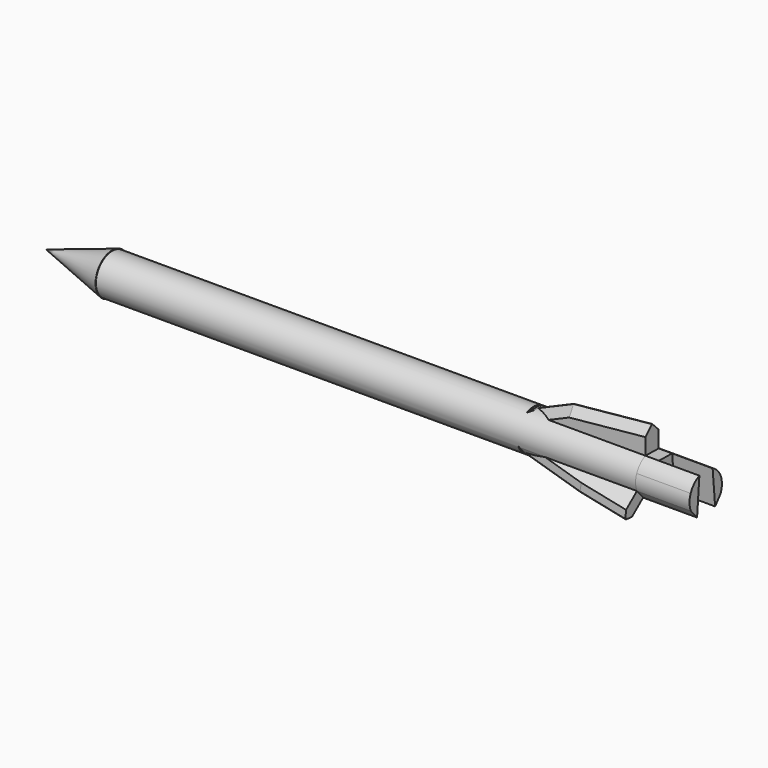
from build123d import *

# Parameters (mm, degrees)
F0_R          = 9.525
F1_DEPTH      = 254
F5_DEPTH      = 55.626
F7_DEPTH      = 6.35
F8_DEPTH      = 25.4
F10_DEPTH     = 25.4
F12_DEPTH     = 25.4
F14_DEPTH     = 25.4
F15_T1_DEPTH  = 44.8533405939
F15_T3_DEPTH  = 44.8533405939
F15_T8_DEPTH  = 28.2795963183
F15_S9_R      = 9.525
F15_T10_DEPTH = 17
F15_T14_DEPTH = 27.9095113127
F15_S15_R     = 9.525
F15_T16_DEPTH = 17
F16_T1_DEPTH  = 52.8359208118
F16_T3_DEPTH  = 52.8359208118
F16_T8_DEPTH  = 31.126263523
F16_S9_R      = 9.525
F16_T10_DEPTH = 18
F16_T14_DEPTH = 35.8525293061
F16_S15_R     = 9.525
F16_T16_DEPTH = 20
F17_T1_DEPTH  = 37.2074314298
F17_T3_DEPTH  = 37.2074314298
F17_T8_DEPTH  = 45.6448991689
F17_S9_R      = 9.525
F17_T10_DEPTH = 25
F17_T14_DEPTH = 44.9174010309
F17_S15_R     = 9.525
F17_T16_DEPTH = 25


# Not quite as in the source:
# - a fillet or chamfer that OpenCascade refuses, or shapes differently, is made with other operations: its cross-section is extruded or revolved along the edge and cut away or added
# - a feature names something its author has since deleted; it is built from what else it names


with BuildPart() as f1:
    # F0 (on Right) → F1 (new body)
    with BuildSketch(Plane.YZ):
        Circle(F0_R)
    extrude(amount=F1_DEPTH)

    # F2 (on Front) → F3 (revolve)
    with BuildSketch(Plane.XZ):
        Polygon((0, -9.7508067265), (0, 0), (-31.0870110989, 0), align=None)
    revolve(axis=Axis((-15.5435055494, 0, 0), (-1, 0, 0)))

    # F4 (on face) → F5 (join)
    with BuildSketch(Plane.YZ.offset(254)):
        with BuildLine():
            ThreePointArc((-3.7328505423, 8.7630731955), (0.1780475173, 9.5233357644), (4.0577948396, 8.6174199178))
            Line((4.0577948396, 8.6174199178), (4.0577948396, 20.311106017))
            Line((4.0577948396, 20.311106017), (-3.7328505423, 20.311106017))
            Line((-3.7328505423, 20.311106017), (-3.7328505423, 8.7630731955))
        make_face()
        with BuildLine():
            ThreePointArc((-5.0939482873, -8.0484356149), (-7.2224802699, -6.2097829069), (-8.7212105654, -3.8296359191))
            Line((-8.7212105654, -3.8296359191), (-17.1272028238, -10.6496075168))
            Line((-17.1272028238, -10.6496075168), (-13.6232364185, -14.9684399422))
            Line((-13.6232364185, -14.9684399422), (-5.0939482873, -8.0484356149))
        make_face()
        with BuildLine():
            Line((13.9740978255, -12.0467544007), (8.7309135752, -3.8074628223))
            ThreePointArc((8.7309135752, -3.8074628223), (7.3970545146, -6.0007674099), (5.5259177996, -7.75821226))
            Line((5.5259177996, -7.75821226), (9.9034377135, -14.6371738298))
            Line((9.9034377135, -14.6371738298), (13.9740978255, -12.0467544007))
        make_face()
    extrude(amount=-F5_DEPTH)

    # F6 (on face) → F7 (join)
    with BuildSketch(Plane.YZ.offset(254)):
        Polygon((4.0577948396, 8.6174199178), (-3.7328505423, 8.7630731955), (-5.0939482873, -8.0484356149), (5.5259177996, -7.75821226), align=None)
        with BuildLine():
            Line((5.5259177996, -7.75821226), (-5.0939482873, -8.0484356149))
            ThreePointArc((-5.0939482873, -8.0484356149), (0.2602053301, -9.5214451732), (5.5259177996, -7.75821226))
        make_face()
    extrude(amount=F7_DEPTH)

    # F6 (on face) → F8 (join)
    with BuildSketch(Plane.YZ.offset(254)):
        Polygon((-5.0939482873, -8.0484356149), (-3.7328505423, 8.7630731955), (-8.8555062097, 3.5079388207), (-8.7212105654, -3.8296359191), align=None)
        Polygon((8.7309135752, 3.8074628223), (4.0577948396, 8.6174199178), (5.5259177996, -7.75821226), (8.7309135752, -3.8074628223), align=None)
        with BuildLine():
            ThreePointArc((9.525, 0), (9.3243653083, 1.9446944743), (8.7309135752, 3.8074628223))
            Line((8.7309135752, 3.8074628223), (8.7309135752, -3.8074628223))
            ThreePointArc((8.7309135752, -3.8074628223), (9.3243653083, -1.9446944743), (9.525, 0))
        make_face()
        with BuildLine():
            ThreePointArc((8.7309135752, 3.8074628223), (6.8316679914, 6.6373140242), (4.0577948396, 8.6174199178))
            Line((4.0577948396, 8.6174199178), (8.7309135752, 3.8074628223))
        make_face()
        with BuildLine():
            Line((-8.7212105654, -3.8296359191), (-8.8555062097, 3.5079388207))
            ThreePointArc((-8.8555062097, 3.5079388207), (-9.5234050588, -0.1743017091), (-8.7212105654, -3.8296359191))
        make_face()
        with BuildLine():
            Line((-8.8555062097, 3.5079388207), (-3.7328505423, 8.7630731955))
            ThreePointArc((-3.7328505423, 8.7630731955), (-6.8206151301, 6.6486716152), (-8.8555062097, 3.5079388207))
        make_face()
    extrude(amount=F8_DEPTH)

    # F9 (on face) → F10 (cut)
    with BuildSketch(Plane(origin=(0, 4.0577948396, 0), x_dir=(-1, 0, 0), z_dir=(0, 1, 0))):
        Polygon((-217.1654254198, 16.6623666883), (-198.374, 8.6174199178), (-198.374, 20.311106017), (-254, 20.311106017), align=None)
    extrude(amount=-F10_DEPTH, mode=Mode.SUBTRACT)

    # F11 (on face) → F12 (cut)
    with BuildSketch(Plane(origin=(0, 4.4898005119, 2.8571450721), x_dir=(-1, 0, 0), z_dir=(0, 0.843661548, 0.5368753975))):
        Polygon((-198.374, -7.8996226746), (-217.1549183124, -14.7158552648), (-254, -17.6657327906), (-198.374, -17.6657327906), align=None)
    extrude(amount=-F12_DEPTH, mode=Mode.SUBTRACT)

    # F13 (on face) → F14 (cut)
    with BuildSketch(Plane(origin=(0, 1.9157700793, -2.3612925984), x_dir=(1, 0, 0), z_dir=(0, 0.6300417268, -0.7765612806))):
        Polygon((230.1693707705, 16.137143597), (254, 20.0100196673), (198.374, 20.0100196673), (198.374, 9.0266132778), align=None)
    extrude(amount=-F14_DEPTH, mode=Mode.SUBTRACT)

    # F15: chamfer of 3.81 on 4 edges, made by hand

    # F15_s2 → F15_t1 (cut)
    with BuildSketch(Plane(origin=(257.4244465349, 0, 25.499811331), x_dir=(0, 1, 0), z_dir=(-0.9951296233, 0, -0.098575011))):
        with BuildLine():
            Line((0.1400317661, 4.7181064364), (4.165557913, 8.7436325833))
            Line((4.165557913, 8.7436325833), (4.241757913, 8.7436325833))
            ThreePointArc((4.241757913, 8.7436325833), (4.1339948396, 6.7847510466), (4.1339948396, 4.8258695099))
            Line((4.1339948396, 4.8258695099), (4.0577948396, 4.7496695099))
            ThreePointArc((4.0577948396, 4.7496695099), (2.0989133028, 4.7496695099), (0.1400317661, 4.6419064364))
            Line((0.1400317661, 4.6419064364), (0.1400317661, 4.7181064364))
        make_face()
    extrude(amount=F15_T1_DEPTH, mode=Mode.SUBTRACT)

    # F15_s4 → F15_t3 (cut)
    with BuildSketch(Plane(origin=(212.789558605, 0, 21.0783927893), x_dir=(0, 1, 0), z_dir=(0.9951296233, 0, 0.098575011))):
        with BuildLine():
            Line((-3.8406136157, -8.7436325833), (0.1849125312, -4.7181064364))
            Line((0.1849125312, -4.7181064364), (0.1849125312, -4.6419064364))
            ThreePointArc((0.1849125312, -4.6419064364), (-1.7739690056, -4.7496695099), (-3.7328505423, -4.7496695099))
            Line((-3.7328505423, -4.7496695099), (-3.8090505423, -4.8258695099))
            ThreePointArc((-3.8090505423, -4.8258695099), (-3.8090505423, -6.7847510466), (-3.9168136157, -8.7436325833))
            Line((-3.9168136157, -8.7436325833), (-3.8406136157, -8.7436325833))
        make_face()
    extrude(amount=F15_T3_DEPTH, mode=Mode.SUBTRACT)


with BuildPart() as f15_tool6:
    # F15_s7 → F15_t8 (new body)
    with BuildSketch(Plane(origin=(193.1590423404, 0, 82.6948557196), x_dir=(0, 1, 0), z_dir=(-0.9192958979, 0, -0.3935670871))):
        with BuildLine():
            Line((0.1400317661, 70.0437554835), (4.165557913, 74.0692816304))
            Line((4.165557913, 74.0692816304), (4.241757913, 74.0692816304))
            ThreePointArc((4.241757913, 74.0692816304), (4.1339948396, 72.1104000937), (4.1339948396, 70.1515185569))
            Line((4.1339948396, 70.1515185569), (4.0577948396, 70.0753185569))
            ThreePointArc((4.0577948396, 70.0753185569), (2.0989133028, 70.0753185569), (0.1400317661, 69.9675554835))
            Line((0.1400317661, 69.9675554835), (0.1400317661, 70.0437554835))
        make_face()
    extrude(amount=F15_T8_DEPTH)

    # F15_s9 → F15_t10 (cut, symmetric)
    with BuildSketch(Plane.YZ.offset(208.5)):
        Circle(F15_S9_R)
    extrude(amount=F15_T10_DEPTH, both=True, mode=Mode.SUBTRACT)


with BuildPart() as f1_1:
    add(f1.part)

    # F15_t5: cut F15_tool6
    add(f15_tool6.part, mode=Mode.SUBTRACT)


with BuildPart() as f15_tool12:
    # F15_s13 → F15_t14 (new body)
    with BuildSketch(Plane(origin=(167.5019430775, 0, 71.7105906496), x_dir=(0, 1, 0), z_dir=(0.9192958979, 0, 0.3935670871))):
        with BuildLine():
            Line((-3.8406136157, -74.0692816304), (0.1849125312, -70.0437554835))
            Line((0.1849125312, -70.0437554835), (0.1849125312, -69.9675554835))
            ThreePointArc((0.1849125312, -69.9675554835), (-1.7739690056, -70.0753185569), (-3.7328505423, -70.0753185569))
            Line((-3.7328505423, -70.0753185569), (-3.8090505423, -70.1515185569))
            ThreePointArc((-3.8090505423, -70.1515185569), (-3.8090505423, -72.1104000937), (-3.9168136157, -74.0692816304))
            Line((-3.9168136157, -74.0692816304), (-3.8406136157, -74.0692816304))
        make_face()
    extrude(amount=F15_T14_DEPTH)

    # F15_s15 → F15_t16 (cut, symmetric)
    with BuildSketch(Plane.YZ.offset(208.7)):
        Circle(F15_S15_R)
    extrude(amount=F15_T16_DEPTH, both=True, mode=Mode.SUBTRACT)


with BuildPart() as f1_2:
    add(f1_1.part)

    # F15_t11: cut F15_tool12
    add(f15_tool12.part, mode=Mode.SUBTRACT)

    # F16: chamfer of 2.286 on 4 edges, made by hand

    # F16_s2 → F16_t1 (cut)
    with BuildSketch(Plane(origin=(259.6477190804, 11.1604697827, -17.5378854343), x_dir=(0.042943471, -0.9990775037, 0), z_dir=(-0.9968103928, -0.0428460235, 0.0673294822))):
        Polygon((2.2434282818, 4.4374187115), (-0.9134913616, 3.7406760293), (1.0133398012, 2.5105875487), align=None)
    extrude(amount=F16_T1_DEPTH, mode=Mode.SUBTRACT)

    # F16_s4 → F16_t3 (cut)
    with BuildSketch(Plane(origin=(206.9803241045, 8.8966606792, -13.980470247), x_dir=(-0.042943471, 0.9990775037, 0), z_dir=(0.9968103928, 0.0428460235, -0.0673294822))):
        Polygon((1.823476661, 7.0337297004), (1.1267339788, 3.8768100571), (3.0535651416, 5.1068985377), align=None)
    extrude(amount=F16_T3_DEPTH, mode=Mode.SUBTRACT)


with BuildPart() as f16_tool6:
    # F16_s7 → F16_t8 (new body)
    with BuildSketch(Plane(origin=(205.9939924457, 40.1379913763, -63.0740020828), x_dir=(0.1912534961, -0.9815406768, 0), z_dir=(-0.9400053053, -0.1831603164, 0.2878234257))):
        Polygon((31.47248323, 51.4536328512), (34.6470195867, 52.0651154105), (33.365492688, 50.1721059525), align=None)
    extrude(amount=F16_T8_DEPTH)

    # F16_s9 → F16_t10 (cut, symmetric)
    with BuildSketch(Plane.YZ.offset(212.3)):
        Circle(F16_S9_R)
    extrude(amount=F16_T10_DEPTH, both=True, mode=Mode.SUBTRACT)


with BuildPart() as f1_3:
    add(f1_2.part)

    # F16_t5: cut F16_tool6
    add(f16_tool6.part, mode=Mode.SUBTRACT)


with BuildPart() as f16_tool12:
    # F16_s13 → F16_t14 (new body)
    with BuildSketch(Plane(origin=(172.2924246879, 33.5712307637, -52.7548042766), x_dir=(-0.1912534961, 0.9815406768, 0), z_dir=(0.9400053053, 0.1831603164, -0.2878234257))):
        Polygon((-30.6515011053, 54.7699959311), (-31.2629836646, 51.5954595744), (-29.3699742066, 52.8769864731), align=None)
    extrude(amount=F16_T14_DEPTH)

    # F16_s15 → F16_t16 (cut, symmetric)
    with BuildSketch(Plane.YZ.offset(210.1)):
        Circle(F16_S15_R)
    extrude(amount=F16_T16_DEPTH, both=True, mode=Mode.SUBTRACT)


with BuildPart() as f1_4:
    add(f1_3.part)

    # F16_t11: cut F16_tool12
    add(f16_tool12.part, mode=Mode.SUBTRACT)

    # F17: chamfer of 2.54 on 4 edges, made by hand

    # F17_s2 → F17_t1 (cut)
    with BuildSketch(Plane(origin=(220.3542251508, -27.8096296574, -22.5625813797), x_dir=(0.1252109944, 0.9921301361, 0), z_dir=(0.9870501192, -0.1245698749, -0.1010663563))):
        Polygon((20.2701864549, 12.3371401962), (16.6998573856, 12.7320456743), (18.2875691812, 10.7494284006), align=None)
    extrude(amount=F17_T1_DEPTH, mode=Mode.SUBTRACT)

    # F17_s4 → F17_t3 (cut)
    with BuildSketch(Plane(origin=(257.0798247798, -32.4445547373, -26.3230009032), x_dir=(-0.1252109944, -0.9921301361, 0), z_dir=(-0.9870501192, 0.1245698749, 0.1010663563))):
        Polygon((-16.7937957885, 16.6782002076), (-16.3988903104, 13.1078711382), (-14.8111785147, 15.090488412), align=None)
    extrude(amount=F17_T3_DEPTH, mode=Mode.SUBTRACT)


with BuildPart() as f17_tool6:
    # F17_s7 → F17_t8 (new body)
    with BuildSketch(Plane(origin=(184.4733137003, -32.036670961, -25.9920755723), x_dir=(0.1711045444, 0.9852528787, 0), z_dir=(0.9758943907, -0.1694792968, -0.1375023858))):
        Polygon((30.9152465813, 20.5992083681), (27.3471595892, 21.0138832013), (28.9238656686, 19.0225022887), align=None)
    extrude(amount=F17_T8_DEPTH)

    # F17_s9 → F17_t10 (cut, symmetric)
    with BuildSketch(Plane.YZ.offset(214.5)):
        Circle(F17_S9_R)
    extrude(amount=F17_T10_DEPTH, both=True, mode=Mode.SUBTRACT)


with BuildPart() as f1_5:
    add(f1_4.part)

    # F17_t5: cut F17_tool6
    add(f17_tool6.part, mode=Mode.SUBTRACT)


with BuildPart() as f17_tool12:
    # F17_s13 → F17_t14 (new body)
    with BuildSketch(Plane(origin=(229.0179147643, -39.7725363756, -32.2683581086), x_dir=(-0.1711045444, -0.9852528787, 0), z_dir=(-0.9758943907, 0.1694792968, 0.1375023858))):
        Polygon((-27.0482787605, 21.3913699029), (-27.4629535937, 24.959456895), (-25.4715726811, 23.3827508156), align=None)
    extrude(amount=F17_T14_DEPTH)

    # F17_s15 → F17_t16 (cut, symmetric)
    with BuildSketch(Plane.YZ.offset(214.9)):
        Circle(F17_S15_R)
    extrude(amount=F17_T16_DEPTH, both=True, mode=Mode.SUBTRACT)


with BuildPart() as f1_6:
    add(f1_5.part)

    # F17_t11: cut F17_tool12
    add(f17_tool12.part, mode=Mode.SUBTRACT)


solid = f1_6.part
